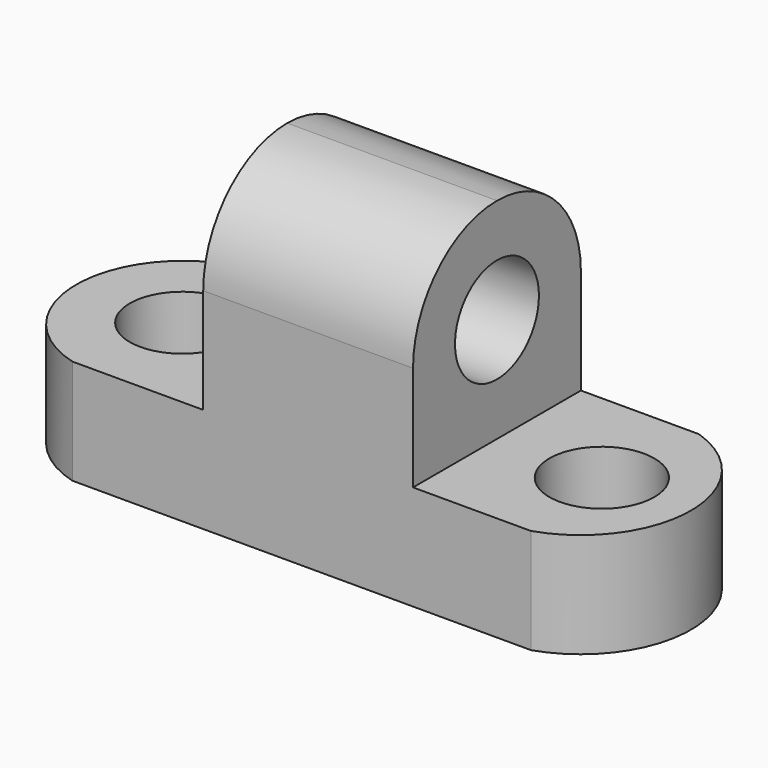
from build123d import *

# Parameters (mm, degrees)
F0_W      = 82.55
F0_H      = 38.1
F1_DEPTH  = 25.4
F2_W      = 28.575
F2_H      = 25.4
F3_DEPTH  = 25.4
F4_R      = 12.69999
F6_DEPTH  = 25.4
F8_DEPTH  = 25.4
F9_R      = 6.35
F10_DEPTH = 25.4
F11_R     = 6.35
F12_DEPTH = 25.4
F13_R     = 6.35
F14_DEPTH = 25.4


# Not quite as in the source:
# - a fillet or chamfer is up to 0.001 mm smaller than in the source, because OpenCascade refuses the exact size
# - a feature names something its author has since deleted; it is built from what else it names


with BuildPart() as f1:
    # F0 (on Front) → F1 (new body)
    with BuildSketch(Plane.XZ):
        with Locations((41.275, 19.05)):
            Rectangle(F0_W, F0_H)
    extrude(amount=F1_DEPTH)

    # F2 (on face) → F3 (cut)
    with BuildSketch(Plane.XZ.offset(25.4)):
        with Locations((14.2875, 25.4)):
            Rectangle(F2_W, F2_H)
        with Locations((68.2625, 25.4)):
            Rectangle(F2_W, F2_H)
    extrude(amount=-F3_DEPTH, mode=Mode.SUBTRACT)

    # F4 (radius 12.7 in the source; OpenCascade refuses exactly that, so slightly less here)
    f4_edges = [f1.edges().sort_by_distance(p)[0] for p in [
        (41.275, 0, 38.1),
        (41.275, -25.4, 38.1),
    ]]
    fillet(f4_edges, radius=F4_R)

    # F5 (on face) → F6 (cut)
    with BuildSketch(Plane.XY.offset(12.7)):
        with BuildLine():
            ThreePointArc((68.2625, 0), (77.4605547287, -12.7), (68.2625, -25.4))
            Line((68.2625, -25.4), (82.55, -25.4))
            Line((82.55, -25.4), (82.55, 0))
            Line((82.55, 0), (68.2625, 0))
        make_face()
    extrude(amount=-F6_DEPTH, mode=Mode.SUBTRACT)

    # F7 (on face) → F8 (cut)
    with BuildSketch(Plane.XY.offset(12.7)):
        with BuildLine():
            ThreePointArc((12.733777985, -25.4), (3.1920308375, -12.0688091081), (14.2875, 0))
            Line((14.2875, 0), (0, 0))
            Line((0, 0), (0, -25.4))
            Line((0, -25.4), (12.733777985, -25.4))
        make_face()
    extrude(amount=-F8_DEPTH, mode=Mode.SUBTRACT)

    # F9 (on face) → F10 (cut)
    with BuildSketch(Plane.XY.offset(12.7)):
        with Locations((66.675, -12.7)):
            Circle(F9_R)
    extrude(amount=-F10_DEPTH, mode=Mode.SUBTRACT)

    # F11 (on face) → F12 (cut)
    with BuildSketch(Plane.XY.offset(12.7)):
        with Locations((15.875, -12.7)):
            Circle(F11_R)
    extrude(amount=-F12_DEPTH, mode=Mode.SUBTRACT)

    # F13 (on face) → F14 (cut)
    with BuildSketch(Plane.YZ.offset(53.975)):
        with Locations((-12.7, 25.4)):
            Circle(F13_R)
    extrude(amount=-F14_DEPTH, mode=Mode.SUBTRACT)


solid = f1.part
